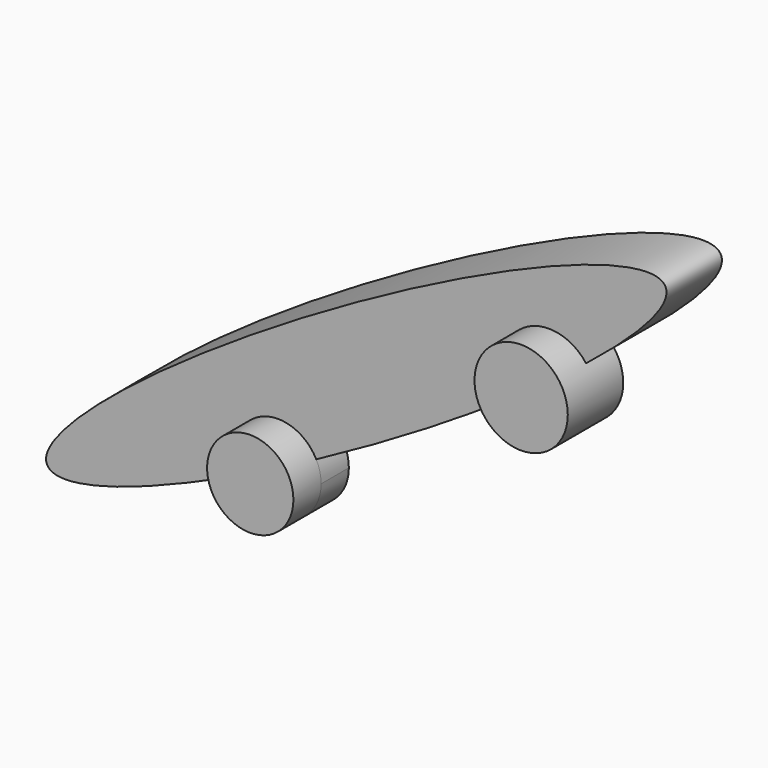
from build123d import *

# Parameters (mm, degrees)
F2_DEPTH = 6.35
F4_R     = 3.9536095432
F4_R_2   = 4.2727196796
F5_DEPTH = 3.175


# Not quite as in the source:
# - the program builds the solid bodies; features that only make, move or delete a surface that nothing else refers to are left out


with BuildPart() as f2:
    # F0 (on Front) → F2 (new body)
    with BuildSketch(Plane.XZ):
        with BuildLine():
            add(Edge.make_bspline(
                [(-9.0637514368, -0.8673357661), (-4.5866868268, -8.5756445749), (35.6313039179, 19.9376927349), (75.8492946625, 48.4510300448), (31.1542393079, 27.6460015438), (-13.5408160468, 6.8409730428), (-9.0637514368, -0.8673357661)],
                knots=[0, 0, 0, 2.0943951024, 2.0943951024, 4.1887902048, 4.1887902048, 6.2831853072, 6.2831853072, 6.2831853072], degree=2, weights=[1, 0.5, 1, 0.5, 1, 0.5, 1]))
        make_face()
    extrude(amount=F2_DEPTH)

    # F4 (on face) → F5 (join, symmetric)
    with BuildSketch(Plane.XZ.offset(6.35)):
        with Locations((12.0665498317, 5.8068699208)):
            Circle(F4_R)
        with Locations((36.886980678, 20.8389717946)):
            Circle(F4_R_2)
    extrude(amount=F5_DEPTH, both=True)


solid = f2.part
